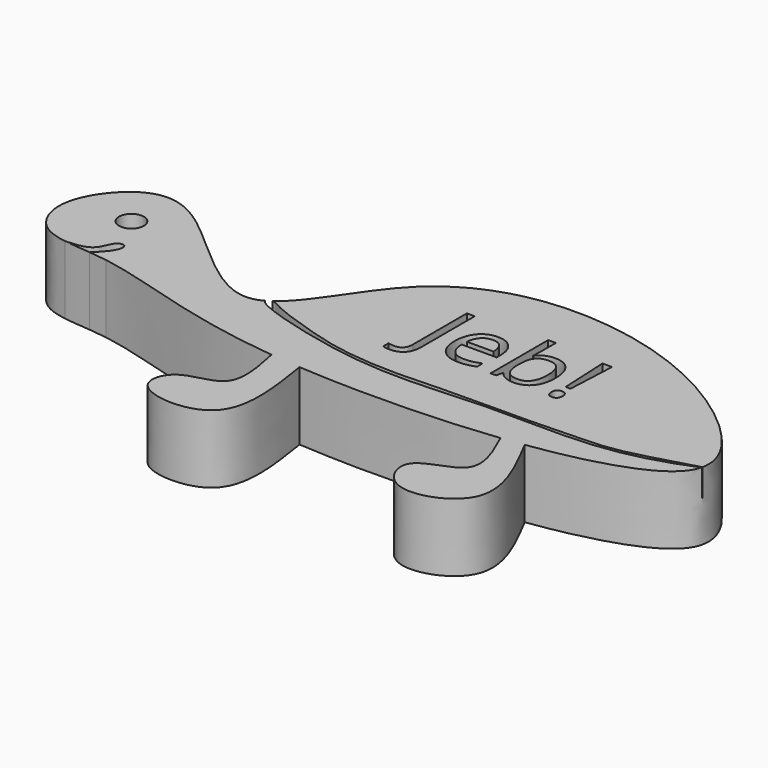
from build123d import *

# Parameters (mm, degrees)
F1_DEPTH     = 6.35
F2_R         = 1.1597285337
F3_DEPTH     = 3.81
F5_DEPTH     = 6.35
F7_DEPTH     = 2.54
F8_TEXT_SIZE = 8.8249690533
F9_DEPTH     = 2.54


# Not quite as in the source:
# - Text() gives the source's letters only with a copy of the font that has no kerning and outlines rounded to 1/6400 em; it was checked with that copy


with BuildPart() as f1:
    # F0 (on Top) → F1 (new body)
    with BuildSketch(Plane.XY):
        with BuildLine():
            add(Edge.make_bspline(
                [(-37.2717380524, -5.1352172159), (-39.8170082525, -4.7361834729), (-43.9606201292, -5.0926873104), (-46.220535145, 0.1843724402), (-42.1119715028, 5.8039183566), (-36.1050175759, 5.3531473416), (-24.4906045717, -8.6996123175), (-18.3117348166, 7.9777012783), (-3.3289954318, 11.3520999104), (11.8243669941, 5.6432752112), (20.5482294827, -4.8885908351), (10.5089927622, -8.0066763966), (4.6908640744, -8.8491633441)],
                knots=[0, 0, 0, 0, 0.067036, 0.1220255105, 0.1860337855, 0.247276073, 0.3441607493, 0.4362155174, 0.5362387877, 0.644937296, 0.7262315995, 0.7963516922, 0.7963516922, 0.7963516922, 0.7963516922], degree=3))
            add(Edge.make_bspline(
                [(-18.553044647, -9.2765223235), (-27.656218744, -8.2981937817), (-32.8667323732, -5.8258102632), (-37.2717380524, -5.1352172159)],
                knots=[0.8839832563, 0.8839832563, 0.8839832563, 0.8839832563, 1, 1, 1, 1], degree=3))
            add(Edge.make_bspline(
                [(-15.7421378398, -9.5230937358), (-16.7112229781, -9.4556967641), (-17.6512350092, -9.3734408377), (-18.553044647, -9.2765223235)],
                knots=[0.8724900105, 0.8724900105, 0.8724900105, 0.8724900105, 0.8839832563, 0.8839832563, 0.8839832563, 0.8839832563], degree=3))
            add(Edge.make_bspline(
                [(2.6502580827, -9.1148757155), (-3.2348474412, -9.8000606421), (-9.9990339947, -9.9225094238), (-15.7421378398, -9.5230937358)],
                knots=[0.8043774147, 0.8043774147, 0.8043774147, 0.8043774147, 0.8724900105, 0.8724900105, 0.8724900105, 0.8724900105], degree=3))
            add(Edge.make_bspline(
                [(4.6908640744, -8.8491633441), (4.0249395875, -8.945591718), (3.343701399, -9.0341402204), (2.6502580827, -9.1148757155)],
                knots=[0.7963516922, 0.7963516922, 0.7963516922, 0.7963516922, 0.8043774147, 0.8043774147, 0.8043774147, 0.8043774147], degree=3))
        make_face()
        with BuildLine():
            add(Edge.make_bspline(
                [(2.6502580827, -9.1148757155), (3.5821342029, -11.1650068297), (5.3410278551, -15.0068268175), (-1.3784620524, -15.5291950427), (1.0761641712, -21.0787299814), (9.4933445294, -18.0324543558), (6.4088620383, -12.1444210888), (4.6908640744, -8.8491633441)],
                knots=[0, 0, 0, 0, 0.19671824, 0.3737540517, 0.534332886, 0.7418593669, 1, 1, 1, 1], degree=3))
            add(Edge.make_bspline(
                [(4.6908640744, -8.8491633441), (4.0249395875, -8.945591718), (3.343701399, -9.0341402204), (2.6502580827, -9.1148757155)],
                knots=[0.7963516922, 0.7963516922, 0.7963516922, 0.7963516922, 0.8043774147, 0.8043774147, 0.8043774147, 0.8043774147], degree=3))
        make_face()
        with BuildLine():
            add(Edge.make_bspline(
                [(-15.7421378398, -9.5230937358), (-16.7112229781, -9.4556967641), (-17.6512350092, -9.3734408377), (-18.553044647, -9.2765223235)],
                knots=[0.8724900105, 0.8724900105, 0.8724900105, 0.8724900105, 0.8839832563, 0.8839832563, 0.8839832563, 0.8839832563], degree=3))
            add(Edge.make_bspline(
                [(-18.553044647, -9.2765223235), (-18.1042030617, -11.454203552), (-17.2785392383, -15.4609027512), (-22.4765920978, -15.257480577), (-23.7255781641, -19.743495076), (-14.0391725685, -20.4123603945), (-15.1311398243, -13.4534930422), (-15.7421378398, -9.5230937358)],
                knots=[0, 0, 0, 0, 0.2019980354, 0.3726808304, 0.5167541631, 0.7310467913, 1, 1, 1, 1], degree=3))
        make_face()
    extrude(amount=F1_DEPTH)

    # F2 (on face) → F3 (cut)
    with BuildSketch(Plane.XY.offset(6.35)):
        with Locations((-39.6432429552, 0.7820653263)):
            Circle(F2_R)
    extrude(amount=-F3_DEPTH, mode=Mode.SUBTRACT)

    # F4 (on face) → F5 (cut)
    with BuildSketch(Plane.XY.offset(6.35)):
        with BuildLine():
            add(Edge.make_bspline(
                [(-41.4465230305, -4.6821867704), (-40.5435892616, -4.6297298162), (-38.8740838202, -4.5275520191), (-38.5449739387, -2.4203569385), (-37.4421257303, -2.4170712758), (-37.6037141853, -3.5874732467), (-38.4516912858, -4.4249150537), (-38.9655673931, -4.9342401461)],
                knots=[0, 0, 0, 0, 0.2578116905, 0.4767787788, 0.6102011886, 0.7636430631, 1, 1, 1, 1], degree=3))
            add(Edge.make_bspline(
                [(-41.4465230305, -4.6821867704), (-40.619537818, -4.7662045623), (-39.7925526056, -4.8502223542), (-38.9655673931, -4.9342401461)],
                knots=[0, 0, 0, 0, 2.4937264844, 2.4937264844, 2.4937264844, 2.4937264844], degree=3))
        make_face()
    extrude(amount=-F5_DEPTH, mode=Mode.SUBTRACT)

    # F6 (on face) → F7 (cut)
    with BuildSketch(Plane.XY.offset(6.35)):
        with BuildLine():
            add(Edge.make_bspline(
                [(-24.228102139, -2.9228765604), (-24.1328674863, -3.6461212944), (-12.0707713334, -7.1385213053), (-1.4665557075, -5.4353851145), (10.0383028272, -6.5068426149), (20.054728814, -2.3966451319), (10.7793271414, -5.4899884492), (7.3085598322, -5.4848725237), (1.9614847297, -5.7477778253), (-4.5867183256, -5.6278205789), (-9.5569740727, -5.9790381492), (-14.5195625376, -5.6615500366), (-18.0679520991, -4.7954501785), (-22.7973371942, -3.195368105), (-23.6381177139, -2.4958805018), (-24.2489827515, -2.7643020018), (-24.228102139, -2.9228765604)],
                knots=[0, 0, 0, 0, 0.1020835433, 0.2109671578, 0.3196268199, 0.3945966148, 0.468654952, 0.5321887842, 0.6017148712, 0.6809776915, 0.7505037799, 0.817502285, 0.878823296, 0.946408133, 0.9776177384, 1, 1, 1, 1], degree=3))
        make_face()
    extrude(amount=-F7_DEPTH, mode=Mode.SUBTRACT)

    # F8 (on face) → F9 (cut)
    with BuildSketch(Plane.XY.offset(6.35)):
        with Locations((-12.3486444354, -1.606528298)):
            Text('Jeb!', F8_TEXT_SIZE, font='Open Sans', text_align=(TextAlign.LEFT, TextAlign.BOTTOM))
    extrude(amount=-F9_DEPTH, mode=Mode.SUBTRACT)


solid = f1.part
